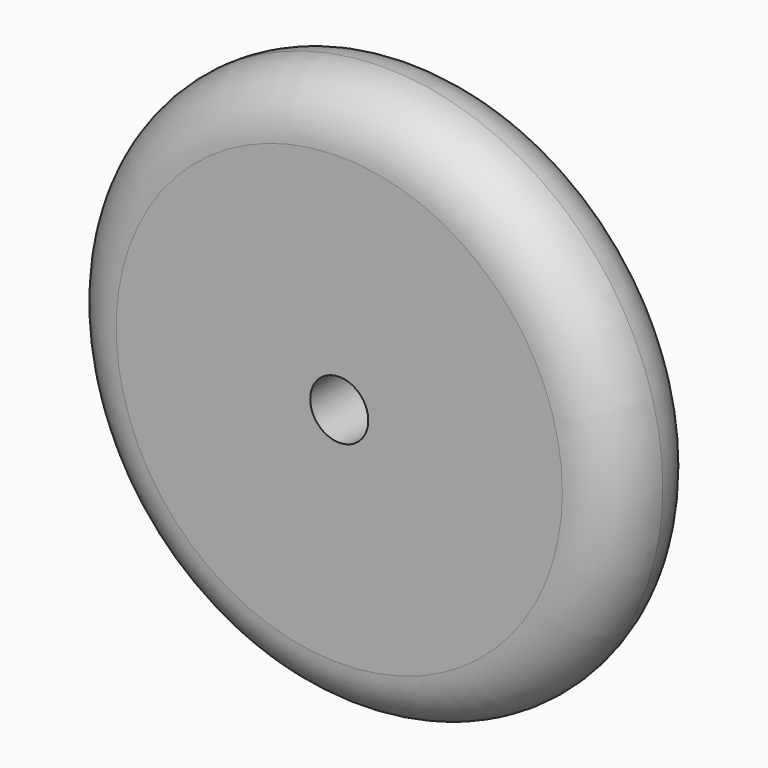
from build123d import *

# Parameters (mm, degrees)
F0_R     = 15.875
F1_DEPTH = 6.35
F3_D     = 3.302
F4_R     = 3.17499


# Not quite as in the source:
# - a fillet or chamfer is up to 0.001 mm smaller than in the source, because OpenCascade refuses the exact size


with BuildPart() as f1:
    # F0 (on Front) → F1 (new body)
    with BuildSketch(Plane.XZ):
        Circle(F0_R)
    extrude(amount=F1_DEPTH)

    # F3 (through all)
    with Locations(Plane.XZ.offset(6.35)):
        with Locations((0, 0)):
            Hole(F3_D / 2)

    # F4 (radius 3.175 in the source; OpenCascade refuses exactly that, so slightly less here)
    f4_edges = [f1.edges().sort_by_distance(p)[0] for p in [
        (-15.875, -6.35, 0),
        (-15.875, 0, 0),
    ]]
    fillet(f4_edges, radius=F4_R)


solid = f1.part
